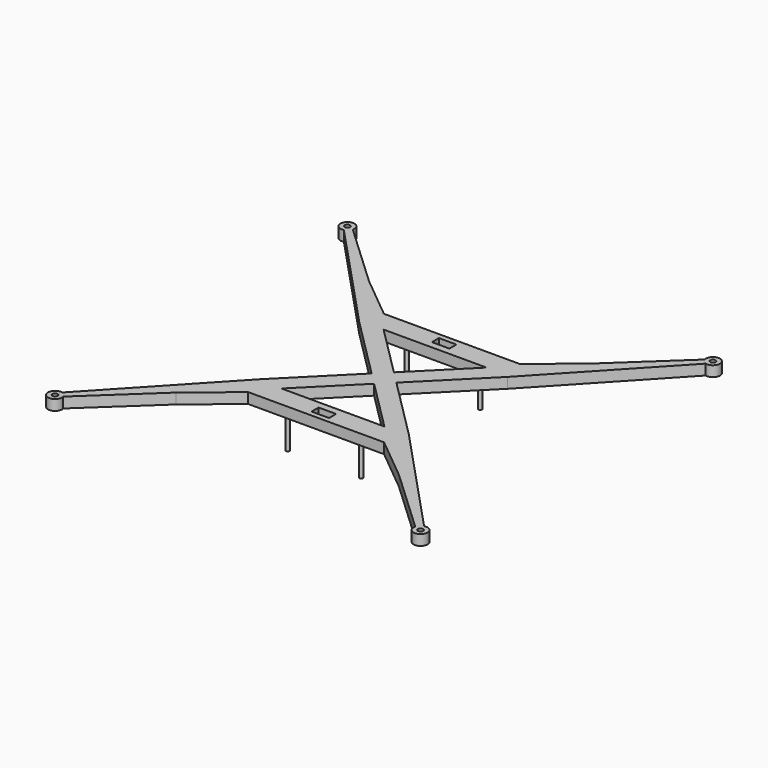
from build123d import *

# Parameters (mm, degrees)
F0_R         = 4
F1_DEPTH     = 6
F3_DEPTH     = 6
F4_R         = 1.5
F5_DEPTH     = 6.001
F6_COUNT     = 4
F8_W         = 85
F8_H         = 12
F9_DEPTH     = 6
F10_R        = 3.55
F10_R_2      = 2.5
F10_W        = 10
F10_H        = 5
F11_DEPTH    = 6.001
F12_C1_SIZE2 = 3
F12_C1_SIZE  = 30
F12_C2_SIZE2 = 30
F12_C2_SIZE  = 3
F12_C3_SIZE2 = 3
F12_C3_SIZE  = 30
F12_C4_SIZE2 = 30
F12_C4_SIZE  = 3
F13_R        = 1
F14_DEPTH    = 20
F15_R        = 3.55
F15_R_2      = 2.5
F16_DEPTH    = 6


# Not quite as in the source:
# - a pattern or mirror of a feature is missing from the dataset's text; its kind, count and spacing are read off the source's solid


with BuildPart() as f1:
    # F0 (on Top) → F1 (new body)
    with BuildSketch(Plane.XY):
        with Locations((-104.5, 104.5)):
            Circle(F0_R)
    extrude(amount=F1_DEPTH)

    # F2 (on Top) → F3 (join, through all)
    with BuildSketch(Plane.XY):
        Polygon((-7.0710678119, 0), (0, 0), (0, 7.0710678119), (-35.3553390593, 42.4264068712), (-100.6362966948, 103.4647238196), (-103.4647238196, 100.6362966948), (-42.4264068712, 35.3553390593), align=None)
    extrude(amount=F3_DEPTH)

    # F4 (on face) → F5 (cut, through all)
    with BuildSketch(Plane.XY.offset(6)):
        with Locations((-104.5, 104.5)):
            Circle(F4_R)
    extrude(amount=-F5_DEPTH, mode=Mode.SUBTRACT)


with BuildPart() as f6_1:
    # F6: instance of F1
    add(f1.part.rotate(Axis((0, 0, 3), (0, 0, -1)), 1 * 360 / F6_COUNT))


with BuildPart() as f6_2:
    # F6: instance of F1
    add(f1.part.rotate(Axis((0, 0, 3), (0, 0, -1)), 2 * 360 / F6_COUNT))


with BuildPart() as f6_3:
    # F6: instance of F1
    add(f1.part.rotate(Axis((0, 0, 3), (0, 0, -1)), 3 * 360 / F6_COUNT))


with BuildPart() as f1_1:
    add(f1.part)

    # F7: union F6_1, F6_2, F6_3
    add(f6_1.part)
    add(f6_2.part)
    add(f6_3.part)

    # F8 (on Top) → F9 (join, through all)
    with BuildSketch(Plane.XY):
        with Locations((0, 42.5)):
            Rectangle(F8_W, F8_H)
    f9 = extrude(amount=F9_DEPTH)

    # F9_copies: F9 across plane
    add(f9.mirror(Plane(origin=(0, 0, 0), x_dir=(0, 0, -1), z_dir=(0, -1, 0))))

    # F10 (on face) → F11 (cut, through all)
    with BuildSketch(Plane.XY.offset(6)):
        with Locations((-21, 42.5)):
            Circle(F10_R)
        with Locations((21, 42.5)):
            Circle(F10_R_2)
        with Locations((0, 43)):
            Rectangle(F10_W, F10_H)
    f11 = extrude(amount=-F11_DEPTH, mode=Mode.SUBTRACT)

    # F11_copies: F11 across plane
    add(f11.mirror(Plane(origin=(0, 0, 0), x_dir=(0, 0, -1), z_dir=(0, -1, 0))), mode=Mode.SUBTRACT)

    # F12: chamfer of 3 x 30 on 4 edges, made by hand

    # F12_c1
    f12_c1_edges = [f1_1.edges().sort_by_distance(p)[0] for p in [
        (-41.8510944399, 48.5, 3),
    ]]
    f12_c1_side = f1_1.faces().sort_by_distance((-41.8949210948, 48.5409783396, 3))[0]
    chamfer(f12_c1_edges, length=F12_C1_SIZE, length2=F12_C1_SIZE2, reference=f12_c1_side)

    # F12_c2
    f12_c2_edges = [f1_1.edges().sort_by_distance(p)[0] for p in [
        (41.8510944399, 48.5, 3),
    ]]
    f12_c2_side = f1_1.faces().sort_by_distance((41.7910944399, 48.5, 3))[0]
    chamfer(f12_c2_edges, length=F12_C2_SIZE, length2=F12_C2_SIZE2, reference=f12_c2_side)

    # F12_c3
    f12_c3_edges = [f1_1.edges().sort_by_distance(p)[0] for p in [
        (41.8510944399, -48.5, 3),
    ]]
    f12_c3_side = f1_1.faces().sort_by_distance((41.8949210948, -48.5409783396, 3))[0]
    chamfer(f12_c3_edges, length=F12_C3_SIZE, length2=F12_C3_SIZE2, reference=f12_c3_side)

    # F12_c4
    f12_c4_edges = [f1_1.edges().sort_by_distance(p)[0] for p in [
        (-41.8510944399, -48.5, 3),
    ]]
    f12_c4_side = f1_1.faces().sort_by_distance((-41.7910944399, -48.5, 3))[0]
    chamfer(f12_c4_edges, length=F12_C4_SIZE, length2=F12_C4_SIZE2, reference=f12_c4_side)



with BuildPart() as f14:
    # F13 (on Top) → F14 (new body)
    with BuildSketch(Plane.XY):
        with Locations((-21, 42.5)):
            Circle(F13_R)
    extrude(amount=-F14_DEPTH)


with BuildPart() as f14b:
    # F13 (on Top) → F14, piece 2 (new body)
    with BuildSketch(Plane.XY):
        with Locations((21, 42.5)):
            Circle(F13_R)
    extrude(amount=-F14_DEPTH)


with BuildPart() as f14c:
    # F13 (on Top) → F14, piece 3 (new body)
    with BuildSketch(Plane.XY):
        with Locations((-21, -42.5)):
            Circle(F13_R)
    extrude(amount=-F14_DEPTH)


with BuildPart() as f14d:
    # F13 (on Top) → F14, piece 4 (new body)
    with BuildSketch(Plane.XY):
        with Locations((21, -42.5)):
            Circle(F13_R)
    extrude(amount=-F14_DEPTH)


with BuildPart() as f1_2:
    add(f1_1.part)

    add(f14.part)  # F16 merges F14

    add(f14b.part)  # F16 merges F14b

    add(f14c.part)  # F16 merges F14c

    add(f14d.part)  # F16 merges F14d
    # F15 (on face) → F16 (join)
    with BuildSketch(Plane.XY.offset(6)):
        with Locations((-21, -42.5)):
            Circle(F15_R)
        with Locations((21, -42.5)):
            Circle(F15_R_2)
        with Locations((21, 42.5)):
            Circle(F15_R_2)
        with Locations((-21, 42.5)):
            Circle(F15_R)
    extrude(amount=-F16_DEPTH)


solid = f1_2.part
